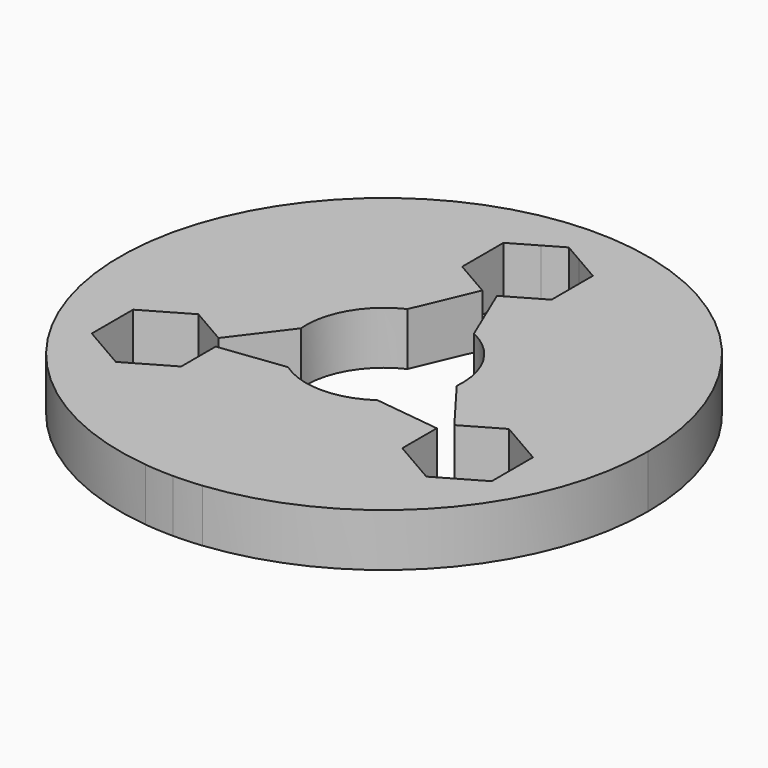
from build123d import *

# Parameters (mm, degrees)
F1_DEPTH = 7.5


# Not quite as in the source:
# - ends of sketch curves that miss each other by under 0.0002 mm in the source are joined


with BuildPart() as f1:
    # F0 (on Top) → F1 (new body)
    with BuildSketch(Plane.XY):
        with BuildLine():
            ThreePointArc((4.0556630512, -37.2800428811), (27.913593144, -25.0415917583), (37.5, 0))
            ThreePointArc((37.5, 0), (-25.0415917583, 27.913593144), (-4.0556630512, -37.2800428811))
            ThreePointArc((-4.0556630512, -37.2800428811), (-2.0308116554, -37.4449703434), (0, -37.5))
            ThreePointArc((0, -37.5), (2.0308116554, -37.4449703434), (4.0556630512, -37.2800428811))
        make_face()
        with BuildLine():
            ThreePointArc((-28.4078604382, -13.2949914876), (-27.1628882386, 15.6825009444), (-2.6901296616, 31.2494245665))
            Line((-2.6901296616, 31.2494245665), (7.92e-08, 32.8025716965))
            Line((7.92e-08, 32.8025716965), (2.6901298478, 31.2494245505))
            ThreePointArc((2.6901298478, 31.2494245505), (23.109946567, 21.2059827173), (31.365001727, 0))
            ThreePointArc((31.365001727, 0), (30.6167921454, -6.8099465531), (28.407860359, -13.2949916568))
            Line((28.407860359, -13.2949916568), (28.407860359, -16.4012859168))
            Line((28.407860359, -16.4012859168), (25.7177305905, -17.9544330629))
            ThreePointArc((25.7177305905, -17.9544330629), (-9.34e-08, -31.365001727), (-25.7177306974, -17.9544329097))
            Line((-25.7177306974, -17.9544329097), (-28.4078604382, -16.4012857797))
            Line((-28.4078604382, -16.4012857797), (-28.4078604382, -13.2949914876))
        make_face(mode=Mode.SUBTRACT)
        with BuildLine():
            ThreePointArc((-11.0725523918, -0.9414030915), (-9.6237073053, 5.5562499901), (-4.7209972243, 10.059813192))
            Line((-4.7209972243, 10.059813192), (-1.0416995056, 18.7393003948))
            Line((-1.0416995056, 18.7393003948), (-6.3499999208, 21.8040490685))
            Line((-6.3499999208, 21.8040490685), (-6.3499999208, 29.1363974872))
            Line((-6.3499999208, 29.1363974872), (-2.6901296616, 31.2494245665))
            ThreePointArc((-2.6901296616, 31.2494245665), (-27.1628882386, 15.6825009444), (-28.4078604382, -13.2949914876))
            Line((-28.4078604382, -13.2949914876), (-28.4078604382, -9.068937361))
            Line((-28.4078604382, -9.068937361), (-22.0578604382, -5.4027631516))
            Line((-22.0578604382, -5.4027631516), (-16.7495600286, -8.467511822))
            Line((-16.7495600286, -8.467511822), (-11.0725523918, -0.9414030915))
        make_face()
        with BuildLine():
            Line((6.3500000792, 21.8040490685), (1.0416996696, 18.739300398))
            Line((1.0416996696, 18.739300398), (4.7209974611, 10.0598130809))
            ThreePointArc((4.7209974611, 10.0598130809), (9.6237072938, 5.5562500099), (11.0725524179, -0.941402785))
            Line((11.0725524179, -0.941402785), (16.7495599439, -8.4675119624))
            Line((16.7495599439, -8.4675119624), (22.057860359, -5.4027632888))
            Line((22.057860359, -5.4027632888), (28.407860359, -9.0689374981))
            Line((28.407860359, -9.0689374981), (28.407860359, -13.2949916568))
            ThreePointArc((28.407860359, -13.2949916568), (30.6167921454, -6.8099465531), (31.365001727, 0))
            ThreePointArc((31.365001727, 0), (23.109946567, 21.2059827173), (2.6901298478, 31.2494245505))
            Line((2.6901298478, 31.2494245505), (6.3500000792, 29.1363974872))
            Line((6.3500000792, 29.1363974872), (6.3500000792, 21.8040490685))
        make_face()
        with BuildLine():
            Line((-6.3515551695, -9.1184101234), (-15.7078604382, -10.2717884324))
            Line((-15.7078604382, -10.2717884324), (-15.7078604382, -16.4012857797))
            Line((-15.7078604382, -16.4012857797), (-22.0578604382, -20.067459989))
            Line((-22.0578604382, -20.067459989), (-25.7177306974, -17.9544329097))
            ThreePointArc((-25.7177306974, -17.9544329097), (-9.34e-08, -31.365001727), (25.7177305905, -17.9544330629))
            Line((25.7177305905, -17.9544330629), (22.057860359, -20.0674601262))
            Line((22.057860359, -20.0674601262), (15.707860359, -16.4012859168))
            Line((15.707860359, -16.4012859168), (15.707860359, -10.271788576))
            Line((15.707860359, -10.271788576), (6.3515549548, -9.118410273))
            ThreePointArc((6.3515549548, -9.118410273), (-1.15e-08, -11.1125), (-6.3515551695, -9.1184101234))
        make_face()
    extrude(amount=F1_DEPTH)


solid = f1.part
